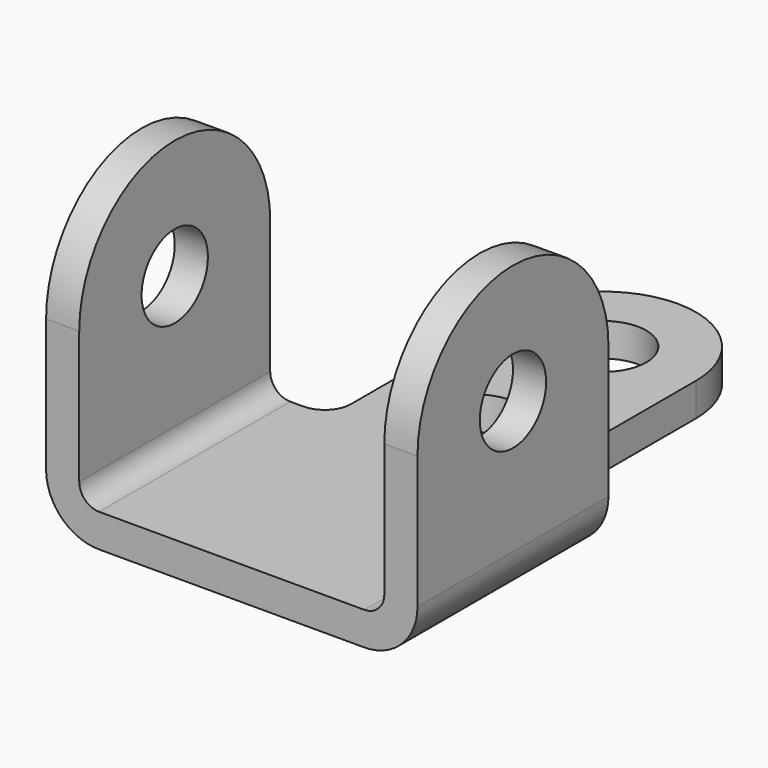
from build123d import *

# Parameters (mm, degrees)
F1_DEPTH = 57.15
F3_DEPTH = 7.93748984
F4_DEPTH = 7.93748984
F6_DEPTH = 7.9375
F7_DEPTH = 7.9375
F8_R     = 10.3251
F9_DEPTH = 7.9375
F10_R    = 6.35


with BuildPart() as f1:
    # F0 (on Front) → F1 (new body)
    with BuildSketch(Plane.XZ):
        with BuildLine():
            Line((-31.75, 0), (0, 0))
            Line((0, 0), (31.75, 0))
            ThreePointArc((31.75, 0), (40.7302561211, 3.7197438789), (44.45, 12.7))
            Line((44.45, 12.7), (44.45, 44.45))
            Line((44.45, 44.45), (36.51251016, 44.4627))
            Line((36.51251016, 44.4627), (36.51251016, 12.7))
            ThreePointArc((36.51251016, 12.7), (35.1176062054, 9.3324039546), (31.75001016, 7.9375))
            Line((31.75001016, 7.9375), (-31.75, 7.9375))
            ThreePointArc((-31.75, 7.9375), (-35.1175960454, 9.3324039546), (-36.5125, 12.7))
            Line((-36.5125, 12.7), (-36.5125, 44.45))
            Line((-36.5125, 44.45), (-44.45, 44.45))
            Line((-44.45, 44.45), (-44.45, 12.7))
            ThreePointArc((-44.45, 12.7), (-40.7302561211, 3.7197438789), (-31.75, 0))
        make_face()
    extrude(amount=F1_DEPTH)

    # F2 (on face) → F3 (join, through all)
    with BuildSketch(Plane.YZ.offset(44.45)):
        with BuildLine():
            ThreePointArc((0, 44.45), (-28.575, 73.025), (-57.15, 44.45))
            Line((-57.15, 44.45), (-38.49751, 44.45))
            ThreePointArc((-38.49751, 44.45), (-28.575, 54.37251), (-18.65249, 44.45))
            Line((-18.65249, 44.45), (0, 44.45))
        make_face()
        with BuildLine():
            ThreePointArc((-18.65249, 44.45), (-28.575, 54.37251), (-38.49751, 44.45))
            ThreePointArc((-38.49751, 44.45), (-28.575, 34.52749), (-18.65249, 44.45))
        make_face()
    extrude(amount=-F3_DEPTH)

    # F2 (on face) → F4 (cut, through all)
    with BuildSketch(Plane.YZ.offset(44.45)):
        with BuildLine():
            Line((-18.65249, 44.45), (-38.49751, 44.45))
            ThreePointArc((-38.49751, 44.45), (-28.575, 34.52749), (-18.65249, 44.45))
        make_face()
        with BuildLine():
            ThreePointArc((-18.65249, 44.45), (-28.575, 54.37251), (-38.49751, 44.45))
            Line((-38.49751, 44.45), (-18.65249, 44.45))
        make_face()
    extrude(amount=-F4_DEPTH, mode=Mode.SUBTRACT)

    # F5 (on face) → F6 (join, through all)
    with BuildSketch(Plane(origin=(-44.45, 0, 0), x_dir=(0, -1, 0), z_dir=(-1, 0, 0))):
        with BuildLine():
            ThreePointArc((57.15, 44.45), (28.575, 73.025), (0, 44.45))
            Line((0, 44.45), (18.65249, 44.45))
            ThreePointArc((18.65249, 44.45), (28.575, 54.37251), (38.49751, 44.45))
            Line((38.49751, 44.45), (57.15, 44.45))
        make_face()
        with BuildLine():
            ThreePointArc((38.49751, 44.45), (28.575, 54.37251), (18.65249, 44.45))
            ThreePointArc((18.65249, 44.45), (28.575, 34.52749), (38.49751, 44.45))
        make_face()
    extrude(amount=-F6_DEPTH)

    # F5 (on face) → F7 (cut, through all)
    with BuildSketch(Plane(origin=(-44.45, 0, 0), x_dir=(0, -1, 0), z_dir=(-1, 0, 0))):
        with BuildLine():
            ThreePointArc((38.49751, 44.45), (28.575, 54.37251), (18.65249, 44.45))
            Line((18.65249, 44.45), (38.49751, 44.45))
        make_face()
        with BuildLine():
            Line((38.49751, 44.45), (18.65249, 44.45))
            ThreePointArc((18.65249, 44.45), (28.575, 34.52749), (38.49751, 44.45))
        make_face()
    extrude(amount=-F7_DEPTH, mode=Mode.SUBTRACT)

    # F8 (on face) → F9 (join, through all)
    with BuildSketch(Plane.XY.offset(7.9375)):
        with BuildLine():
            ThreePointArc((22.225, 53.975), (0, 76.2), (-22.225, 53.975))
            Line((-22.225, 53.975), (-22.225, 0))
            Line((-22.225, 0), (22.225, 0))
            Line((22.225, 0), (22.225, 53.975))
        make_face()
        with Locations((0, 15.875)):
            Circle(F8_R, mode=Mode.SUBTRACT)
        with Locations((0, 53.975)):
            Circle(F8_R, mode=Mode.SUBTRACT)
    extrude(amount=-F9_DEPTH)

    # F10
    f10_edges = [f1.edges().sort_by_distance(p)[0] for p in [
        (22.225, 0, 3.96875),
        (-22.225, 0, 3.96875),
    ]]
    fillet(f10_edges, radius=F10_R)


solid = f1.part
